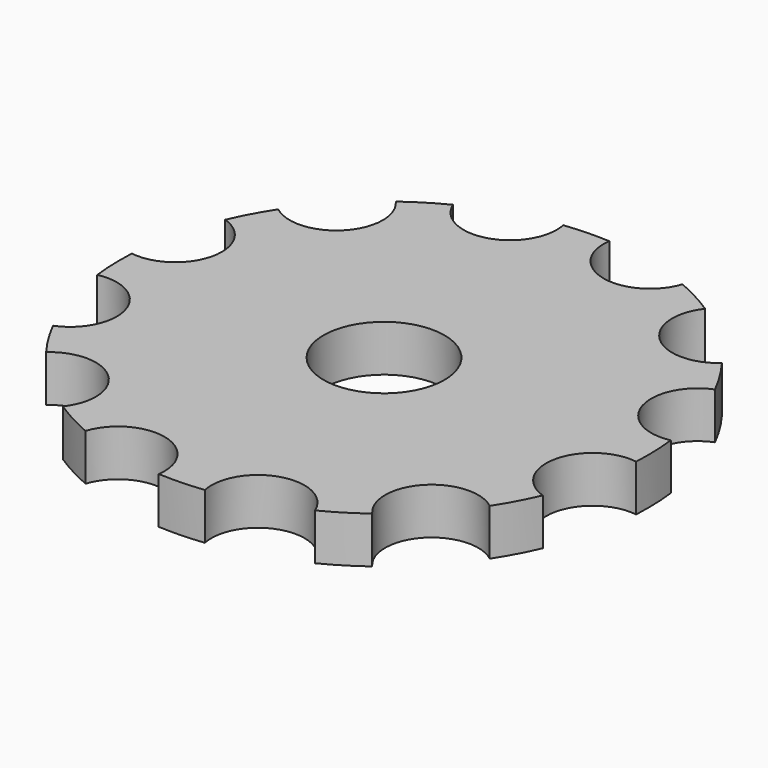
from build123d import *

# Parameters (mm, degrees)
F0_R     = 11.35
F1_DEPTH = 2
F2_R     = 2.6
F3_DEPTH = 25


# Not quite as in the source:
# - a feature names something its author has since deleted; it is built from what else it names


with BuildPart() as f1:
    # F0 (on Top) → F1 (new body)
    with BuildSketch(Plane.XY):
        Circle(F0_R)
    extrude(amount=F1_DEPTH)

    # F2 (on face) → F3 (cut)
    with BuildSketch(Plane.XY.offset(2)):
        with BuildLine():
            ThreePointArc((9.1045560576, 6.7771350137), (7.7736409673, 8.2700064155), (6.2013506213, 9.506090178))
            ThreePointArc((6.2013506213, 9.506090178), (6.4038363916, 6.8127365625), (9.1045560576, 6.7771350137))
        make_face()
        with BuildLine():
            ThreePointArc((9.1045560576, 6.7771350137), (9.5987204424, 7.4520303097), (9.7736409673, 8.2700064155))
            ThreePointArc((9.7736409673, 8.2700064155), (8.4276361156, 10.1600567709), (6.2013506213, 9.506090178))
            ThreePointArc((6.2013506213, 9.506090178), (7.7736409673, 8.2700064155), (9.1045560576, 6.7771350137))
        make_face()
        with BuildLine():
            ThreePointArc((0.6174820868, 11.3331908954), (2.1395167155, 9.1019211282), (4.4962093293, 10.4214491155))
            ThreePointArc((4.4962093293, 10.4214491155), (2.5971673498, 11.0488561289), (0.6174820868, 11.3331908954))
        make_face()
        with BuildLine():
            ThreePointArc((0.6174820868, 11.3331908954), (2.5971673498, 11.0488561289), (4.4962093293, 10.4214491155))
            ThreePointArc((4.4962093293, 10.4214491155), (4.5717665445, 10.73111721), (4.5971673498, 11.0488561289))
            ThreePointArc((4.5971673498, 11.0488561289), (2.7396971257, 13.04377098), (0.6174820868, 11.3331908954))
        make_face()
        with BuildLine():
            ThreePointArc((-5.1318402741, 10.1235722648), (-3.2752151616, 10.8671737653), (-1.3168930579, 11.2733443429))
            ThreePointArc((-1.3168930579, 11.2733443429), (-3.8523455866, 12.7820942526), (-5.1318402741, 10.1235722648))
        make_face()
        with BuildLine():
            ThreePointArc((-1.2752151616, 10.8671737653), (-1.2856619194, 11.0713254155), (-1.3168930579, 11.2733443429))
            ThreePointArc((-1.3168930579, 11.2733443429), (-3.2752151616, 10.8671737653), (-5.1318402741, 10.1235722648))
            ThreePointArc((-5.1318402741, 10.1235722648), (-2.8965663963, 8.9033445689), (-1.2752151616, 10.8671737653))
        make_face()
        with BuildLine():
            ThreePointArc((-9.506090178, 6.2013506213), (-8.2700064155, 7.7736409673), (-6.7771350137, 9.1045560576))
            ThreePointArc((-6.7771350137, 9.1045560576), (-9.7272762684, 9.143445543), (-9.506090178, 6.2013506213))
        make_face()
        with BuildLine():
            ThreePointArc((-6.2700064155, 7.7736409673), (-6.4010838912, 8.4857705891), (-6.7771350137, 9.1045560576))
            ThreePointArc((-6.7771350137, 9.1045560576), (-8.2700064155, 7.7736409673), (-9.506090178, 6.2013506213))
            ThreePointArc((-9.506090178, 6.2013506213), (-7.3959833966, 5.97472914), (-6.2700064155, 7.7736409673))
        make_face()
        with BuildLine():
            ThreePointArc((-11.3331908954, 0.6174820868), (-11.0488561289, 2.5971673498), (-10.4214491155, 4.4962093293))
            ThreePointArc((-10.4214491155, 4.4962093293), (-12.9957911296, 3.0548179842), (-11.3331908954, 0.6174820868))
        make_face()
        with BuildLine():
            ThreePointArc((-9.0488561289, 2.5971673498), (-9.427928304, 3.7687444863), (-10.4214491155, 4.4962093293))
            ThreePointArc((-10.4214491155, 4.4962093293), (-11.0488561289, 2.5971673498), (-11.3331908954, 0.6174820868))
            ThreePointArc((-11.3331908954, 0.6174820868), (-9.7390220808, 1.0857657597), (-9.0488561289, 2.5971673498))
        make_face()
        with BuildLine():
            ThreePointArc((11.2733443429, 1.3168930579), (10.8671737653, 3.2752151616), (10.1235722648, 5.1318402741))
            ThreePointArc((10.1235722648, 5.1318402741), (8.952253278, 2.6980847366), (11.2733443429, 1.3168930579))
        make_face()
        with BuildLine():
            ThreePointArc((12.8671737653, 3.2752151616), (11.9880655975, 4.9315972131), (10.1235722648, 5.1318402741))
            ThreePointArc((10.1235722648, 5.1318402741), (10.8671737653, 3.2752151616), (11.2733443429, 1.3168930579))
            ThreePointArc((11.2733443429, 1.3168930579), (12.4183573707, 2.0127455887), (12.8671737653, 3.2752151616))
        make_face()
        with BuildLine():
            ThreePointArc((10.4214491155, -4.4962093293), (11.0488561289, -2.5971673498), (11.3331908954, -0.6174820868))
            ThreePointArc((11.3331908954, -0.6174820868), (9.1019211282, -2.1395167155), (10.4214491155, -4.4962093293))
        make_face()
        with BuildLine():
            ThreePointArc((13.0488561289, -2.5971673498), (12.560257719, -1.2873333018), (11.3331908954, -0.6174820868))
            ThreePointArc((11.3331908954, -0.6174820868), (11.0488561289, -2.5971673498), (10.4214491155, -4.4962093293))
            ThreePointArc((10.4214491155, -4.4962093293), (12.2204332653, -4.2180951747), (13.0488561289, -2.5971673498))
        make_face()
        with BuildLine():
            ThreePointArc((-4.4962093293, -10.4214491155), (-3.0548179842, -12.9957911296), (-0.6174820868, -11.3331908954))
            ThreePointArc((-0.6174820868, -11.3331908954), (-2.5971673498, -11.0488561289), (-4.4962093293, -10.4214491155))
        make_face()
        with BuildLine():
            ThreePointArc((-4.4962093293, -10.4214491155), (-2.5971673498, -11.0488561289), (-0.6174820868, -11.3331908954))
            ThreePointArc((-0.6174820868, -11.3331908954), (-0.6022524988, -11.1913859047), (-0.5971673498, -11.0488561289))
            ThreePointArc((-0.5971673498, -11.0488561289), (-2.2794284309, -9.0742569343), (-4.4962093293, -10.4214491155))
        make_face()
        with BuildLine():
            ThreePointArc((-10.1235722648, -5.1318402741), (-10.8671737653, -3.2752151616), (-11.2733443429, -1.3168930579))
            ThreePointArc((-11.2733443429, -1.3168930579), (-12.7820942526, -3.8523455866), (-10.1235722648, -5.1318402741))
        make_face()
        with BuildLine():
            ThreePointArc((-8.8671737653, -3.2752151616), (-9.6047041924, -1.7240315562), (-11.2733443429, -1.3168930579))
            ThreePointArc((-11.2733443429, -1.3168930579), (-10.8671737653, -3.2752151616), (-10.1235722648, -5.1318402741))
            ThreePointArc((-10.1235722648, -5.1318402741), (-9.2107917138, -4.3961069938), (-8.8671737653, -3.2752151616))
        make_face()
        with BuildLine():
            ThreePointArc((-6.2013506213, -9.506090178), (-7.7736409673, -8.2700064155), (-9.1045560576, -6.7771350137))
            ThreePointArc((-9.1045560576, -6.7771350137), (-9.143445543, -9.7272762684), (-6.2013506213, -9.506090178))
        make_face()
        with BuildLine():
            ThreePointArc((-5.7736409673, -8.2700064155), (-6.9556648615, -6.4449269404), (-9.1045560576, -6.7771350137))
            ThreePointArc((-9.1045560576, -6.7771350137), (-7.7736409673, -8.2700064155), (-6.2013506213, -9.506090178))
            ThreePointArc((-6.2013506213, -9.506090178), (-5.8835906119, -8.9240015638), (-5.7736409673, -8.2700064155))
        make_face()
        with BuildLine():
            ThreePointArc((6.7771350137, -9.1045560576), (8.2700064155, -7.7736409673), (9.506090178, -6.2013506213))
            ThreePointArc((9.506090178, -6.2013506213), (6.8127365625, -6.4038363916), (6.7771350137, -9.1045560576))
        make_face()
        with BuildLine():
            ThreePointArc((10.2700064155, -7.7736409673), (10.0689182428, -6.8996179484), (9.506090178, -6.2013506213))
            ThreePointArc((9.506090178, -6.2013506213), (8.2700064155, -7.7736409673), (6.7771350137, -9.1045560576))
            ThreePointArc((6.7771350137, -9.1045560576), (8.9821360372, -9.6425634916), (10.2700064155, -7.7736409673))
        make_face()
        with BuildLine():
            ThreePointArc((1.3168930579, -11.2733443429), (3.2752151616, -10.8671737653), (5.1318402741, -10.1235722648))
            ThreePointArc((5.1318402741, -10.1235722648), (2.6980847366, -8.952253278), (1.3168930579, -11.2733443429))
        make_face()
        with BuildLine():
            ThreePointArc((5.2752151616, -10.8671737653), (5.239044358, -10.488525), (5.1318402741, -10.1235722648))
            ThreePointArc((5.1318402741, -10.1235722648), (3.2752151616, -10.8671737653), (1.3168930579, -11.2733443429))
            ThreePointArc((1.3168930579, -11.2733443429), (3.4793668118, -12.8567270075), (5.2752151616, -10.8671737653))
        make_face()
        Circle(F2_R)
    extrude(amount=-F3_DEPTH, mode=Mode.SUBTRACT)


solid = f1.part
